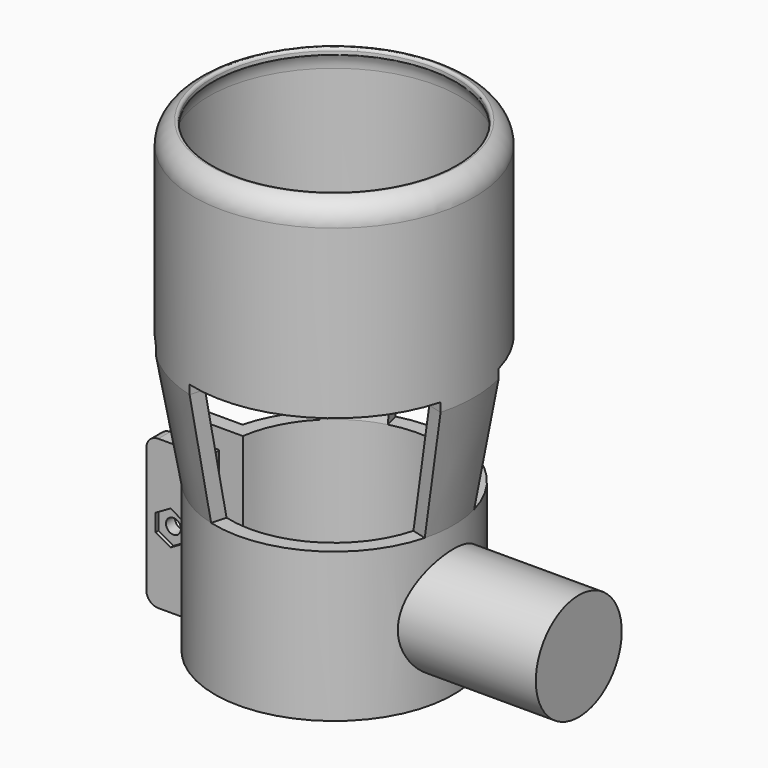
from build123d import *

# Parameters (mm, degrees)
F0_W           = 3.175
F0_H           = 38.1
F1_ANGLE_BACK  = 15
F1_ANGLE       = 30
F0_H_2         = 15.875
F0_H_3         = 11.43
F0_H_4         = 4.445
F0_W_2         = 3.9863166107
F0_H_5         = 1.4520821328
F5_COUNT       = 3
F5_ANGLE       = 240
F6_DEPTH       = 6.35
F0_W_3         = 17.383622241
F0_H_6         = 31.75
F7_DEPTH       = 3.175
F9_D           = 3.175
F9_CBORE_D     = 6.35
F9_CBORE_DEPTH = 0.508
F10_R          = 1.5875
F11_DEPTH      = 0.762
F13_R          = 0.508
F15_T2_ANGLE   = 90
F15_T4_ANGLE   = 90
F15_T6_ANGLE   = 90
F0_W_4         = 26.67


# Not quite as in the source:
# - a fillet or chamfer that OpenCascade refuses, or shapes differently, is made with other operations: its cross-section is extruded or revolved along the edge and cut away or added


with BuildPart() as f1:
    # F0 (on Front) → F1 (revolve)
    with BuildSketch(Plane.XZ, mode=Mode.PRIVATE) as f1_sk:
        with Locations((28.2575, 60.325)):
            Rectangle(F0_W, F0_H)
    revolve(f1_sk.sketch.rotate(Axis((0, 0, 31.75), (0, 0, -1)), -F1_ANGLE_BACK), axis=Axis((0, 0, 31.75), (0, 0, -1)), revolution_arc=F1_ANGLE)



with BuildPart() as f1b:
    # F0 (on Front) → F1, piece 2 (revolve)
    with BuildSketch(Plane.XZ, mode=Mode.PRIVATE) as f1_sk:
        with Locations((23.8125, -7.9375)):
            Rectangle(F0_W, F0_H_2)
        with Locations((23.8125, 5.715)):
            Rectangle(F0_W, F0_H_3)
        with Locations((23.8125, 13.6525)):
            Rectangle(F0_W, F0_H_4)
    revolve(f1_sk.sketch.rotate(Axis((0, 0, 31.75), (0, 0, -1)), -F1_ANGLE_BACK), axis=Axis((0, 0, 31.75), (0, 0, -1)), revolution_arc=F1_ANGLE)


with BuildPart() as f1_1:
    add(f1.part)

    add(f1b.part)  # F2 merges F1b
    # F1_face (on face) → F2 section 0
    with BuildSketch(Plane(origin=(27.9652046604, 0, 41.275), x_dir=(1, 0, 0), z_dir=(0, 0, -1))):
        with BuildLine():
            ThreePointArc((-2.2039628732, 6.9027039329), (-1.2952046604, 0), (-2.2039628732, -6.9027039329))
            Line((-2.2039628732, -6.9027039329), (0.8628516252, -7.7244544011))
            ThreePointArc((0.8628516252, -7.7244544011), (1.8797953396, 0), (0.8628516252, 7.7244544011))
            Line((0.8628516252, 7.7244544011), (-2.2039628732, 6.9027039329))
        make_face()
    # F1_face1 (on face) → F2 section 1
    with BuildSketch(Plane(origin=(23.5762929935, 0, 15.875), x_dir=(1, 0, 0), z_dir=(0, 0, 1))):
        with BuildLine():
            ThreePointArc((0.9582229943, -6.5740037456), (1.8237070065, 0), (0.9582229943, 6.5740037456))
            Line((0.9582229943, 6.5740037456), (-2.1085915042, 5.7522532774))
            ThreePointArc((-2.1085915042, 5.7522532774), (-1.3512929935, 0), (-2.1085915042, -5.7522532774))
            Line((-2.1085915042, -5.7522532774), (0.9582229943, -6.5740037456))
        make_face()
    loft()

    # F0 (on Front) → F3 (revolve)
    with BuildSketch(Plane.XZ):
        with Locations((28.2575, 60.325)):
            Rectangle(F0_W, F0_H)
        with Locations((23.8125, -7.9375)):
            Rectangle(F0_W, F0_H_2)
        with Locations((23.8125, 5.715)):
            Rectangle(F0_W, F0_H_3)
        with Locations((23.8125, 13.6525)):
            Rectangle(F0_W, F0_H_4)
        with BuildLine():
            ThreePointArc((25.8586833893, 82.3102101397), (26.4634380154, 80.8976369566), (26.67, 79.375))
            Line((26.67, 79.375), (29.845, 79.375))
            Line((29.845, 79.375), (29.845, 82.3102101397))
            Line((29.845, 82.3102101397), (25.8586833893, 82.3102101397))
        make_face()
        with Locations((27.8518416946, 83.0362512061)):
            Rectangle(F0_W_2, F0_H_5)
    revolve(axis=Axis((0, 0, 31.75), (0, 0, -1)))

    # F4: union 


with BuildPart() as f5_1:
    # F5: instance of F1
    add(f1_1.part.rotate(Axis((0, 0, 31.75), (0, 0, -1)), 1 * F5_ANGLE / (F5_COUNT - 1)))


with BuildPart() as f5_2:
    # F5: instance of F1
    add(f1_1.part.rotate(Axis((0, 0, 31.75), (0, 0, -1)), 2 * F5_ANGLE / (F5_COUNT - 1)))


with BuildPart() as f1_2:
    add(f1_1.part)

    add(f5_1.part)  # F6 merges F5_1

    add(f5_2.part)  # F6 merges F5_2
    # F0 (on Front) → F6 (join, symmetric)
    with BuildSketch(Plane.XZ):
        with BuildLine():
            Line((-32.385, -15.875), (-22.225, -15.875))
            Line((-22.225, -15.875), (-22.225, 15.875))
            Line((-22.225, 15.875), (-32.385, 15.875))
            ThreePointArc((-32.385, 15.875), (-34.1810512242, 15.1310512242), (-34.925, 13.335))
            Line((-34.925, 13.335), (-34.925, -13.335))
            ThreePointArc((-34.925, -13.335), (-34.1810512242, -15.1310512242), (-32.385, -15.875))
        make_face()
    extrude(amount=F6_DEPTH, both=True)

    # F0 (on Front) → F7 (cut, symmetric)
    with BuildSketch(Plane.XZ):
        with BuildLine():
            Line((-4.841377759, -29.4260326773), (-4.841377759, -15.875))
            Line((-4.841377759, -15.875), (-22.225, -15.875))
            Line((-22.225, -15.875), (-32.385, -15.875))
            ThreePointArc((-32.385, -15.875), (-34.1810512242, -15.1310512242), (-34.925, -13.335))
            Line((-34.925, -13.335), (-34.925, 13.335))
            ThreePointArc((-34.925, 13.335), (-34.1810512242, 15.1310512242), (-32.385, 15.875))
            Line((-32.385, 15.875), (-22.225, 15.875))
            Line((-22.225, 15.875), (-4.841377759, 15.875))
            Line((-4.841377759, 15.875), (-4.841377759, 29.4260326773))
            Line((-4.841377759, 29.4260326773), (-39.608622241, 29.4260326773))
            Line((-39.608622241, 29.4260326773), (-39.608622241, -29.4260326773))
            Line((-39.608622241, -29.4260326773), (-4.841377759, -29.4260326773))
        make_face()
        with Locations((-13.5331888795, 0)):
            Rectangle(F0_W_3, F0_H_6)
        with BuildLine():
            Line((-32.385, -15.875), (-22.225, -15.875))
            Line((-22.225, -15.875), (-22.225, 15.875))
            Line((-22.225, 15.875), (-32.385, 15.875))
            ThreePointArc((-32.385, 15.875), (-34.1810512242, 15.1310512242), (-34.925, 13.335))
            Line((-34.925, 13.335), (-34.925, -13.335))
            ThreePointArc((-34.925, -13.335), (-34.1810512242, -15.1310512242), (-32.385, -15.875))
        make_face()
    extrude(amount=F7_DEPTH, both=True, mode=Mode.SUBTRACT)

    # F9 (through all)
    with Locations(Plane(origin=(0, 6.35, 0), x_dir=(-1, 0, 0), z_dir=(0, 1, 0))):
        with Locations((29.7592221242, 0)):
            CounterBoreHole(F9_D / 2, F9_CBORE_D / 2, F9_CBORE_DEPTH)

    # F10 (on face) → F11 (cut)
    with BuildSketch(Plane.XZ.offset(6.35)):
        Polygon((-29.7592221242, -3.6661742094), (-26.5842221242, -1.8330871047), (-26.5842221242, 1.8330871047), (-29.7592221242, 3.6661742094), (-32.9342221242, 1.8330871047), (-32.9342221242, -1.8330871047), align=None)
        with Locations((-29.7592221242, 0)):
            Circle(F10_R, mode=Mode.SUBTRACT)
    extrude(amount=-F11_DEPTH, mode=Mode.SUBTRACT)

    # F12: fillet of radius 5.08 on 1 edges, made by hand

    # F12_s1 → F12_t2 (revolve, cut)
    with BuildSketch(Plane(origin=(0, 0, 0), x_dir=(0, 0, 1), z_dir=(-0.8660254038, -0.5, 0))):
        with BuildLine():
            ThreePointArc((83.7622922724, 25.8586833893), (81.9834385897, 28.7249439149), (78.8014197036, 29.845))
            Line((78.8014197036, 29.845), (83.7622922724, 29.845))
            Line((83.7622922724, 29.845), (83.7622922724, 25.8586833893))
        make_face()
    revolve(axis=Axis((0, 0, 83.7622922724), (0, 0, -1)), mode=Mode.SUBTRACT)

    # F13
    f13_edges = [f1_2.edges().sort_by_distance(p)[0] for p in [
        (12.929342, -22.394277, 83.762292),
    ]]
    fillet(f13_edges, radius=F13_R)

    # F14: union 

    # F15: chamfer of 5.08 on 3 edges, made by hand

    # F15_s1 → F15_t2 (revolve, cut)
    with BuildSketch(Plane(origin=(0, 0, 0), x_dir=(0, 0, 1), z_dir=(0.7071067812, -0.7071067812, 0))):
        Polygon((41.275, 31.75), (46.355, 26.67), (41.275, 26.67), align=None)
    revolve(axis=Axis((0, 0, 41.275), (0, 0, -1)), revolution_arc=F15_T2_ANGLE, mode=Mode.SUBTRACT)

    # F15_s3 → F15_t4 (revolve, cut)
    with BuildSketch(Plane(origin=(0, 0, 0), x_dir=(0, 0, 1), z_dir=(0.2588190451, 0.9659258263, 0))):
        Polygon((41.275, 31.75), (46.355, 26.67), (41.275, 26.67), align=None)
    revolve(axis=Axis((0, 0, 41.275), (0, 0, -1)), revolution_arc=F15_T4_ANGLE, mode=Mode.SUBTRACT)

    # F15_s5 → F15_t6 (revolve, cut)
    with BuildSketch(Plane(origin=(0, 0, 0), x_dir=(0, 0, 1), z_dir=(-0.9659258263, -0.2588190451, 0))):
        Polygon((41.275, 31.75), (46.355, 26.67), (41.275, 26.67), align=None)
    revolve(axis=Axis((0, 0, 41.275), (0, 0, -1)), revolution_arc=F15_T6_ANGLE, mode=Mode.SUBTRACT)

    # F0 (on Front) → F16 (revolve)
    with BuildSketch(Plane.XZ):
        with Locations((38.735, 5.715)):
            Rectangle(F0_W_4, F0_H_3)
        with Locations((23.8125, 5.715)):
            Rectangle(F0_W, F0_H_3)
    revolve(axis=Axis((38.735, 0, 0), (-1, 0, 0)))


solid = f1_2.part
